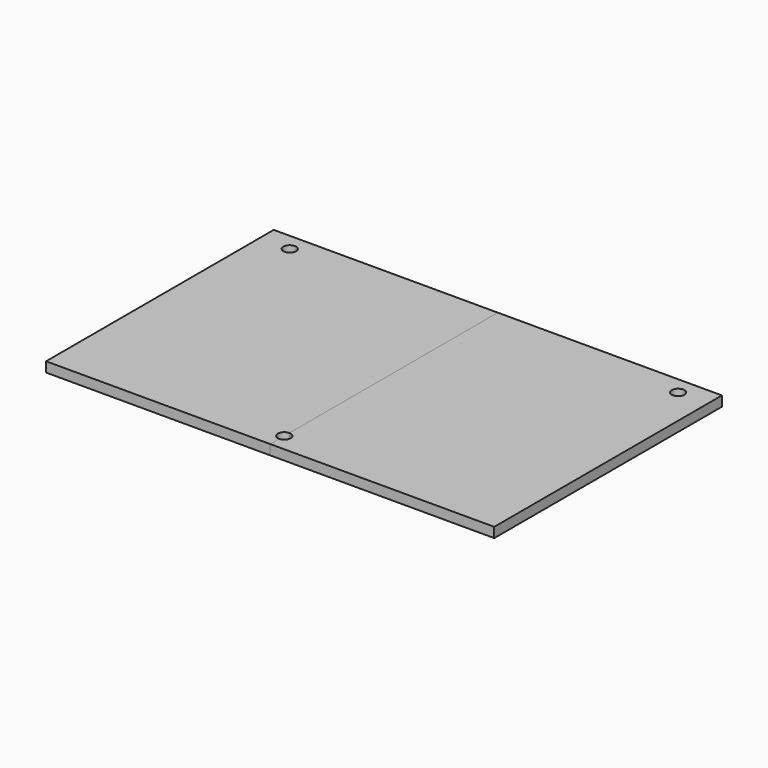
from build123d import *
from build123d import SkipClean  # not in build123d's __all__

# Parameters (mm, degrees)
F0_R     = 2.775
F0_R_2   = 1.275
F1_DEPTH = 2


with BuildPart() as f1:
    # F0 (on Top) → F1 (new body)
    with BuildSketch(Plane.XY):
        with BuildLine():
            Line((0, 28.575), (-45, 28.575))
            Line((-45, 28.575), (-45, -28.575))
            Line((-45, -28.575), (0, -28.575))
            Line((0, -28.575), (0, -27.8123737215))
            ThreePointArc((0, -27.8123737215), (-2.775, -25.0373737215), (0, -22.2623737215))
            Line((0, -22.2623737215), (0, 28.575))
        make_face()
        with Locations((-39, 25.075)):
            Circle(F0_R, mode=Mode.SUBTRACT)
        with BuildLine():
            Line((0, -23.7623737215), (0, -22.2623737215))
            ThreePointArc((0, -22.2623737215), (-2.775, -25.0373737215), (0, -27.8123737215))
            Line((0, -27.8123737215), (0, -26.3123737215))
            ThreePointArc((0, -26.3123737215), (-1.275, -25.0373737215), (0, -23.7623737215))
        make_face()
        with Locations((-39, 25.075)):
            Circle(F0_R)
        with Locations((-39, 25.075)):
            Circle(F0_R_2, mode=Mode.SUBTRACT)
    extrude(amount=F1_DEPTH)

    # F2: F1 across face


with BuildPart() as f1_1:
    add(f1.part, clean=False)
    with SkipClean():  # cleaning this boolean's faces spoils the solid; the shape is the same uncleaned
        add(f1.part.mirror(Plane(origin=(0, 2.4063131393, 1), x_dir=(0, 1, 0), z_dir=(1, 0, 0))), clean=False)


solid = f1_1.part
